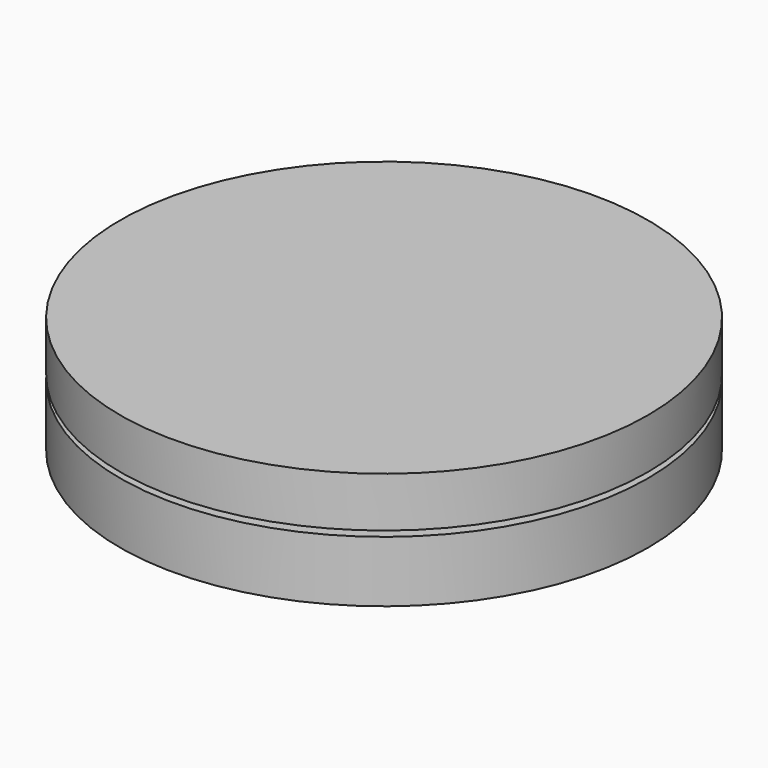
from build123d import *

# Parameters (mm, degrees)
F0_R      = 47.5
F0_R_2    = 5.5
F1_DEPTH  = 2.5
F2_W      = 26.6
F2_H      = 11.5
F3_DEPTH  = 1.5
F4_R      = 1.25
F5_DEPTH  = 4.001
F6_R      = 5.5
F7_DEPTH  = 5
F9_DEPTH  = 4
F11_W     = 30
F11_H     = 14
F12_DEPTH = 9
F10_W     = 24
F10_H     = 8
F13_DEPTH = 7.5
F14_W     = 16
F14_H     = 8
F14_R     = 1
F15_DEPTH = 4.001
F17_W     = 15.5
F17_H     = 56
F18_DEPTH = 13
F16_W     = 11.5
F16_H     = 50
F19_DEPTH = 13
F21_W     = 11.5
F21_H     = 2
F20_W     = 11.5
F20_H     = 2
F22_DEPTH = 2.501
F23_W     = 11.5
F23_H     = 2
F24_DEPTH = 75.501
F25_W     = 11.5
F25_H     = 2
F26_DEPTH = 75.501
F27_W     = 11
F27_H     = 12.5
F28_DEPTH = 6
F29_DEPTH = 2.501
F30_R     = 47.5
F30_R_2   = 44.5
F31_DEPTH = 8.5
F32_R     = 45.5
F32_R_2   = 44.5
F33_DEPTH = 3
F34_R     = 2.5
F34_R_2   = 1.25
F35_DEPTH = 1.5
F37_R     = 47.5
F38_DEPTH = 1.5
F39_R     = 47.5
F39_R_2   = 44.5
F40_DEPTH = 4.5
F41_R     = 47.5
F41_R_2   = 46.5
F42_DEPTH = 3
F43_R     = 5
F43_R_2   = 1.8
F44_DEPTH = 4
F45_DEPTH = 1


with BuildPart() as f1:
    # F0 (on Top) → F1 (new body)
    with BuildSketch(Plane.XY):
        Circle(F0_R)
        Circle(F0_R_2, mode=Mode.SUBTRACT)
    extrude(amount=F1_DEPTH)

    # F2 (on face) → F3 (join)
    with BuildSketch(Plane.XY.offset(2.5)):
        with Locations((0, -24.25)):
            Rectangle(F2_W, F2_H)
    extrude(amount=F3_DEPTH)

    # F4 (on face) → F5 (cut, through all)
    with BuildSketch(Plane.XY.offset(4)):
        with Locations((-9, -22.75)):
            Circle(F4_R)
        with Locations((9, -22.75)):
            Circle(F4_R)
    extrude(amount=-F5_DEPTH, mode=Mode.SUBTRACT)

    # F6 (on face) → F7 (join)
    with BuildSketch(Plane.XY.offset(2.5)):
        with BuildLine():
            Line((-6.6143782777, -7.5), (6.6143782777, -7.5))
            ThreePointArc((6.6143782777, -7.5), (0, 10), (-6.6143782777, -7.5))
        make_face()
        Circle(F6_R, mode=Mode.SUBTRACT)
    extrude(amount=F7_DEPTH)

    # F8 (on face) → F9 (join)
    with BuildSketch(Plane.XY.offset(7.5)):
        with BuildLine():
            Line((1, -7.5), (6.6143782777, -7.5))
            ThreePointArc((6.6143782777, -7.5), (0, 10), (-6.6143782777, -7.5))
            Line((-6.6143782777, -7.5), (-1, -7.5))
            Line((-1, -7.5), (-1, -6.4226162893))
            ThreePointArc((-1, -6.4226162893), (0, 6.5), (1, -6.4226162893))
            Line((1, -6.4226162893), (1, -7.5))
        make_face()
    extrude(amount=F9_DEPTH)

    # F11 (on face) → F12 (join)
    with BuildSketch(Plane.XY.offset(2.5)):
        with Locations((0, 20)):
            Rectangle(F11_W, F11_H)
    extrude(amount=F12_DEPTH)

    # F10 (on face) → F13 (cut)
    with BuildSketch(Plane(origin=(0, 0, 0), x_dir=(1, 0, 0), z_dir=(0, 0, -1))):
        with Locations((0, -20)):
            Rectangle(F10_W, F10_H)
    extrude(amount=-F13_DEPTH, mode=Mode.SUBTRACT)

    # F14 (on face) → F15 (cut, through all)
    with BuildSketch(Plane(origin=(0, 0, 7.5), x_dir=(1, 0, 0), z_dir=(0, 0, -1))):
        with Locations((0, -20)):
            Rectangle(F14_W, F14_H)
        with Locations((-9.5, -20)):
            Circle(F14_R)
        with Locations((9.5, -20)):
            Circle(F14_R)
    extrude(amount=-F15_DEPTH, mode=Mode.SUBTRACT)

    # F17 (on face) → F18 (join)
    with BuildSketch(Plane.XY.offset(2.5)):
        with Locations((-22.5, 0)):
            Rectangle(F17_W, F17_H)
        with Locations((22.5, 0)):
            Rectangle(F17_W, F17_H)
    extrude(amount=F18_DEPTH)

    # F16 (on face) → F19 (cut)
    with BuildSketch(Plane(origin=(0, 0, 0), x_dir=(1, 0, 0), z_dir=(0, 0, -1))):
        with Locations((-22.5, 0)):
            Rectangle(F16_W, F16_H)
        with Locations((22.5, 0)):
            Rectangle(F16_W, F16_H)
    extrude(amount=-F19_DEPTH, mode=Mode.SUBTRACT)

    # F21 (on face) + F20 (on face) → F22 (cut, through all)
    with BuildSketch(Plane(origin=(0, 0, 13), x_dir=(1, 0, 0), z_dir=(0, 0, -1))):
        with Locations((-22.5, 24)):
            Rectangle(F21_W, F21_H)
        with Locations((-22.5, -24)):
            Rectangle(F21_W, F21_H)
    with BuildSketch(Plane(origin=(0, 0, 13), x_dir=(1, 0, 0), z_dir=(0, 0, -1))):
        with Locations((22.5, -24)):
            Rectangle(F20_W, F20_H)
        with Locations((22.5, 24)):
            Rectangle(F20_W, F20_H)
    extrude(amount=-F22_DEPTH, mode=Mode.SUBTRACT)

    # F23 (on face) → F24 (cut, through all)
    with BuildSketch(Plane.XZ.offset(28)):
        with Locations((22.5, 3.5)):
            Rectangle(F23_W, F23_H)
    extrude(amount=-F24_DEPTH, mode=Mode.SUBTRACT)

    # F25 (on face) → F26 (cut, through all)
    with BuildSketch(Plane.XZ.offset(28)):
        with Locations((-22.5, 3.5)):
            Rectangle(F25_W, F25_H)
    extrude(amount=-F26_DEPTH, mode=Mode.SUBTRACT)

    # F27 (on face) → F28 (join)
    with BuildSketch(Plane.XY.offset(2.5)):
        with Locations((0, 33.25)):
            Rectangle(F27_W, F27_H)
        with BuildLine():
            Line((-3.5, 32.5), (-3.5, 37.5))
            Line((-3.5, 37.5), (3.5, 37.5))
            Line((3.5, 37.5), (3.5, 32.5))
            ThreePointArc((3.5, 32.5), (0, 29), (-3.5, 32.5))
        make_face(mode=Mode.SUBTRACT)
    extrude(amount=F28_DEPTH)

    # F29 (cut, through all): a face of the model
    f29_faces = [f1.faces().sort_by_distance(p)[0] for p in [
        (0, 33.5861765733, 2.5),
    ]]
    extrude(f29_faces, amount=-F29_DEPTH, mode=Mode.SUBTRACT)

    # F30 (on face) → F31 (join)
    with BuildSketch(Plane.XY.offset(2.5)):
        Circle(F30_R)
        Circle(F30_R_2, mode=Mode.SUBTRACT)
    extrude(amount=F31_DEPTH)

    # F32 (on face) → F33 (join)
    with BuildSketch(Plane.XY.offset(11)):
        Circle(F32_R)
        Circle(F32_R_2, mode=Mode.SUBTRACT)
    extrude(amount=F33_DEPTH)

    # F34 (on face) → F35 (cut)
    with BuildSketch(Plane(origin=(0, 0, 0), x_dir=(1, 0, 0), z_dir=(0, 0, -1))):
        with Locations((-9, 22.75)):
            Circle(F34_R)
        with Locations((-9, 22.75)):
            Circle(F34_R_2, mode=Mode.SUBTRACT)
        with Locations((9, 22.75)):
            Circle(F34_R)
        with Locations((9, 22.75)):
            Circle(F34_R_2, mode=Mode.SUBTRACT)
        with Locations((9, 22.75)):
            Circle(F34_R_2)
        with Locations((-9, 22.75)):
            Circle(F34_R_2)
    extrude(amount=-F35_DEPTH, mode=Mode.SUBTRACT)


with BuildPart() as f38:
    # F37 (on offset) → F38 (new body)
    with BuildSketch(Plane.XY.offset(21)):
        Circle(F37_R)
    extrude(amount=-F38_DEPTH)

    # F39 (on face) → F40 (join)
    with BuildSketch(Plane(origin=(0, 0, 19.5), x_dir=(1, 0, 0), z_dir=(0, 0, -1))):
        Circle(F39_R)
        Circle(F39_R_2, mode=Mode.SUBTRACT)
    extrude(amount=F40_DEPTH)

    # F41 (on face) → F42 (join)
    with BuildSketch(Plane(origin=(0, 0, 15), x_dir=(1, 0, 0), z_dir=(0, 0, -1))):
        Circle(F41_R)
        Circle(F41_R_2, mode=Mode.SUBTRACT)
    extrude(amount=F42_DEPTH)

    # F43 (on face) → F44 (join)
    with BuildSketch(Plane(origin=(0, 0, 19.5), x_dir=(1, 0, 0), z_dir=(0, 0, -1))):
        Circle(F43_R)
        Circle(F43_R_2, mode=Mode.SUBTRACT)
    extrude(amount=F44_DEPTH)

    # F45 (cut): a face of the model
    f45_faces = [f38.faces().sort_by_distance(p)[0] for p in [
        (0, 0, 19.5),
    ]]
    extrude(f45_faces, amount=-F45_DEPTH, mode=Mode.SUBTRACT)


solid = Compound([f1.part, f38.part])
